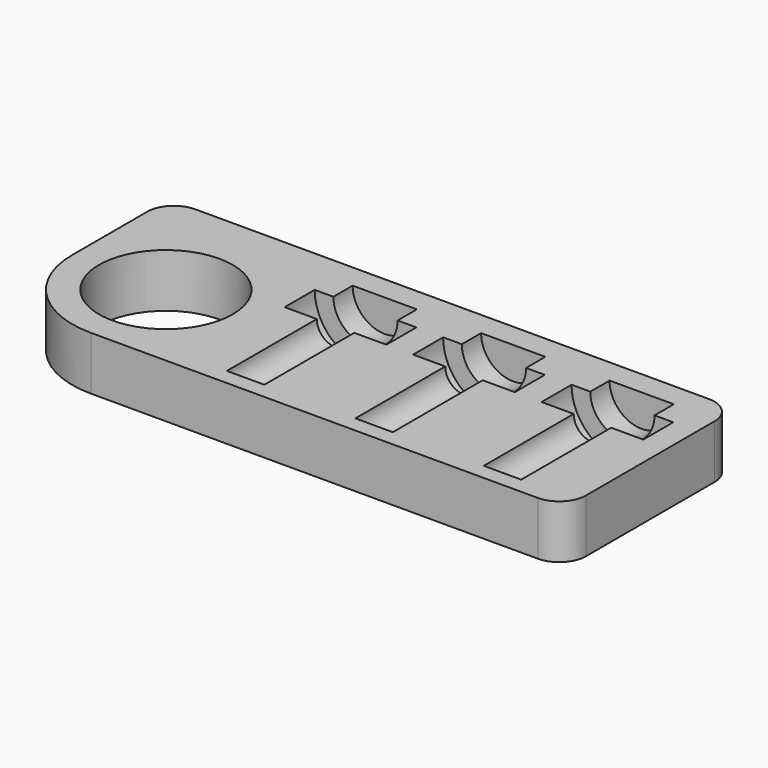
from build123d import *

# Parameters (mm, degrees)
F0_R         = 12.5
F1_DEPTH     = 10
F6_TEXT_SIZE = 5.5555555556
F7_DEPTH     = 1


# Not quite as in the source:
# - Text() gives the source's letters only with a copy of the font that has no kerning and outlines rounded to 1/6400 em; it was checked with that copy


with BuildPart() as f1:
    # F0 (on Top) → F1 (new body)
    with BuildSketch(Plane.XY):
        with BuildLine():
            ThreePointArc((0, 17.5), (5.1256313292, 5.1256313292), (17.5, 0))
            Line((17.5, 0), (101, 0))
            ThreePointArc((101, 0), (104.5355339059, 1.4644660941), (106, 5))
            Line((106, 5), (106, 35))
            ThreePointArc((106, 35), (104.5355339059, 38.5355339059), (101, 40))
            Line((101, 40), (5, 40))
            ThreePointArc((5, 40), (1.4644660941, 38.5355339059), (0, 35))
            Line((0, 35), (0, 17.5))
        make_face()
        with Locations((17.5, 17.5)):
            Circle(F0_R, mode=Mode.SUBTRACT)
    extrude(amount=F1_DEPTH)

    # F2 (on face) → F3 (revolve, cut)
    with BuildSketch(Plane.XY.offset(10)):
        Polygon((44, 24), (44, 3), (47.5, 3), (47.5, 24), (53.5, 24), (53.5, 31), (50, 31), (50, 35.5), (44, 35.5), (44, 31), align=None)
    revolve(axis=Axis((44, 13.5, 10), (0, 1, 0)), mode=Mode.SUBTRACT)

    # F2 (on face) → F4 (revolve, cut)
    with BuildSketch(Plane.XY.offset(10)):
        Polygon((68, 24), (68, 3), (71.5, 3), (71.5, 24), (77.5, 24), (77.5, 31), (74, 31), (74, 35.5), (68, 35.5), (68, 31), align=None)
    revolve(axis=Axis((68, 13.5, 10), (0, 1, 0)), mode=Mode.SUBTRACT)

    # F2 (on face) → F5 (revolve, cut)
    with BuildSketch(Plane.XY.offset(10)):
        Polygon((92, 24), (92, 3), (95.5, 3), (95.5, 24), (101.5, 24), (101.5, 31), (98, 31), (98, 35.5), (92, 35.5), (92, 31), align=None)
    revolve(axis=Axis((92, 13.5, 10), (0, 1, 0)), mode=Mode.SUBTRACT)

    # F6 (on face) → F7 (cut)
    with BuildSketch(Plane(origin=(0, 0, 0), x_dir=(1, 0, 0), z_dir=(0, 0, -1))):
        with Locations((30, -9)):
            Text('990', F6_TEXT_SIZE, font='Open Sans', text_align=(TextAlign.LEFT, TextAlign.BOTTOM))
    extrude(amount=-F7_DEPTH, mode=Mode.SUBTRACT)


solid = f1.part
